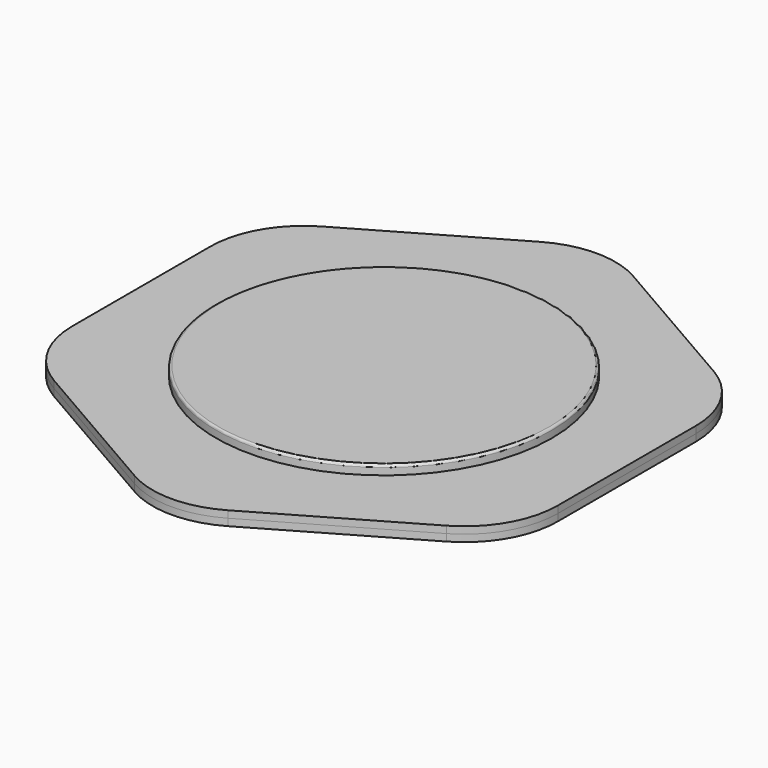
from build123d import *

# Parameters (mm, degrees)
F0_R      = 457.2
F1_DEPTH  = 6.35
F2_R      = 457.2
F2_R_2    = 12.7
F2_R_3    = 3.175
F2_R_4    = 74.6125
F3_DEPTH  = 19.05
F4_R      = 457.2
F4_R_2    = 12.7
F4_R_3    = 3.175
F4_R_4    = 15.875
F5_DEPTH  = 19.05
F6_R      = 74.6125
F6_R_2    = 3.175
F6_R_3    = 58.7375
F7_DEPTH  = 3.175
F9_R      = 457.2
F10_DEPTH = 19.05
F11_R     = 6.34999


# Not quite as in the source:
# - a fillet or chamfer is up to 0.001 mm smaller than in the source, because OpenCascade refuses the exact size


with BuildPart() as f1:
    # F0 (on Top) → F1 (new body)
    with BuildSketch(Plane.XY):
        Circle(F0_R)
    extrude(amount=-F1_DEPTH)

    # F11 (radius 6.35 in the source; OpenCascade refuses exactly that, so slightly less here)
    f11_edges = [f1.edges().sort_by_distance(p)[0] for p in [
        (-457.2, 0, 0),
    ]]
    fillet(f11_edges, radius=F11_R)


with BuildPart() as f3:
    # F2 (on face) → F3 (new body)
    with BuildSketch(Plane(origin=(0, 0, -6.35), x_dir=(1, 0, 0), z_dir=(0, 0, -1))):
        Circle(F2_R)
        with Locations((-291.8583239347, -291.8583239347)):
            Circle(F2_R_2, mode=Mode.SUBTRACT)
        with Locations((-260.427427511, -260.427427511)):
            Circle(F2_R_2, mode=Mode.SUBTRACT)
        with Locations((-228.9965310873, -228.9965310873)):
            Circle(F2_R_2, mode=Mode.SUBTRACT)
        with Locations((-157.9525867087, -381.331277044)):
            Circle(F2_R_3, mode=Mode.SUBTRACT)
        with Locations((-381.331277044, -157.9525867087)):
            Circle(F2_R_3, mode=Mode.SUBTRACT)
        with Locations((-197.5656346635, -197.5656346635)):
            Circle(F2_R_2, mode=Mode.SUBTRACT)
        with Locations((-166.1347382398, -166.1347382398)):
            Circle(F2_R_2, mode=Mode.SUBTRACT)
        with Locations((-134.703841816, -134.703841816)):
            Circle(F2_R_2, mode=Mode.SUBTRACT)
        with Locations((-103.2729453923, -103.2729453923)):
            Circle(F2_R_2, mode=Mode.SUBTRACT)
        with Locations((-71.8420489686, -71.8420489686)):
            Circle(F2_R_2, mode=Mode.SUBTRACT)
        with Locations((0, -412.75)):
            Circle(F2_R_2, mode=Mode.SUBTRACT)
        with Locations((0, -368.3)):
            Circle(F2_R_2, mode=Mode.SUBTRACT)
        with Locations((157.9525867087, -381.331277044)):
            Circle(F2_R_3, mode=Mode.SUBTRACT)
        with Locations((0, -323.85)):
            Circle(F2_R_2, mode=Mode.SUBTRACT)
        with Locations((0, -279.4)):
            Circle(F2_R_2, mode=Mode.SUBTRACT)
        with Locations((0, -234.95)):
            Circle(F2_R_2, mode=Mode.SUBTRACT)
        with Locations((291.8583239347, -291.8583239347)):
            Circle(F2_R_2, mode=Mode.SUBTRACT)
        with Locations((260.427427511, -260.427427511)):
            Circle(F2_R_2, mode=Mode.SUBTRACT)
        with Locations((228.9965310873, -228.9965310873)):
            Circle(F2_R_2, mode=Mode.SUBTRACT)
        with Locations((0, -190.5)):
            Circle(F2_R_2, mode=Mode.SUBTRACT)
        with Locations((0, -146.05)):
            Circle(F2_R_2, mode=Mode.SUBTRACT)
        with Locations((197.5656346635, -197.5656346635)):
            Circle(F2_R_2, mode=Mode.SUBTRACT)
        with Locations((166.1347382398, -166.1347382398)):
            Circle(F2_R_2, mode=Mode.SUBTRACT)
        with Locations((134.703841816, -134.703841816)):
            Circle(F2_R_2, mode=Mode.SUBTRACT)
        with Locations((0, -101.6)):
            Circle(F2_R_2, mode=Mode.SUBTRACT)
        with Locations((103.2729453923, -103.2729453923)):
            Circle(F2_R_2, mode=Mode.SUBTRACT)
        with Locations((71.8420489686, -71.8420489686)):
            Circle(F2_R_2, mode=Mode.SUBTRACT)
        with Locations((381.331277044, -157.9525867087)):
            Circle(F2_R_3, mode=Mode.SUBTRACT)
        with Locations((-412.75, 0)):
            Circle(F2_R_2, mode=Mode.SUBTRACT)
        with Locations((-368.3, 0)):
            Circle(F2_R_2, mode=Mode.SUBTRACT)
        with Locations((-323.85, 0)):
            Circle(F2_R_2, mode=Mode.SUBTRACT)
        with Locations((-279.4, 0)):
            Circle(F2_R_2, mode=Mode.SUBTRACT)
        with Locations((-234.95, 0)):
            Circle(F2_R_2, mode=Mode.SUBTRACT)
        with Locations((-381.331277044, 157.9525867087)):
            Circle(F2_R_3, mode=Mode.SUBTRACT)
        with Locations((-190.5, 0)):
            Circle(F2_R_2, mode=Mode.SUBTRACT)
        with Locations((-146.05, 0)):
            Circle(F2_R_2, mode=Mode.SUBTRACT)
        with Locations((-101.6, 0)):
            Circle(F2_R_2, mode=Mode.SUBTRACT)
        with Locations((-71.8420489686, 71.8420489686)):
            Circle(F2_R_2, mode=Mode.SUBTRACT)
        with Locations((-103.2729453923, 103.2729453923)):
            Circle(F2_R_2, mode=Mode.SUBTRACT)
        with Locations((-134.703841816, 134.703841816)):
            Circle(F2_R_2, mode=Mode.SUBTRACT)
        with Locations((-166.1347382398, 166.1347382398)):
            Circle(F2_R_2, mode=Mode.SUBTRACT)
        with Locations((-197.5656346635, 197.5656346635)):
            Circle(F2_R_2, mode=Mode.SUBTRACT)
        with Locations((-228.9965310873, 228.9965310873)):
            Circle(F2_R_2, mode=Mode.SUBTRACT)
        with Locations((-260.427427511, 260.427427511)):
            Circle(F2_R_2, mode=Mode.SUBTRACT)
        with Locations((-291.8583239347, 291.8583239347)):
            Circle(F2_R_2, mode=Mode.SUBTRACT)
        with Locations((-157.9525867087, 381.331277044)):
            Circle(F2_R_3, mode=Mode.SUBTRACT)
        Circle(F2_R_4, mode=Mode.SUBTRACT)
        with Locations((101.6, 0)):
            Circle(F2_R_2, mode=Mode.SUBTRACT)
        with Locations((0, 101.6)):
            Circle(F2_R_2, mode=Mode.SUBTRACT)
        with Locations((71.8420489686, 71.8420489686)):
            Circle(F2_R_2, mode=Mode.SUBTRACT)
        with Locations((103.2729453923, 103.2729453923)):
            Circle(F2_R_2, mode=Mode.SUBTRACT)
        with Locations((146.05, 0)):
            Circle(F2_R_2, mode=Mode.SUBTRACT)
        with Locations((190.5, 0)):
            Circle(F2_R_2, mode=Mode.SUBTRACT)
        with Locations((0, 146.05)):
            Circle(F2_R_2, mode=Mode.SUBTRACT)
        with Locations((0, 190.5)):
            Circle(F2_R_2, mode=Mode.SUBTRACT)
        with Locations((134.703841816, 134.703841816)):
            Circle(F2_R_2, mode=Mode.SUBTRACT)
        with Locations((166.1347382398, 166.1347382398)):
            Circle(F2_R_2, mode=Mode.SUBTRACT)
        with Locations((197.5656346635, 197.5656346635)):
            Circle(F2_R_2, mode=Mode.SUBTRACT)
        with Locations((234.95, 0)):
            Circle(F2_R_2, mode=Mode.SUBTRACT)
        with Locations((279.4, 0)):
            Circle(F2_R_2, mode=Mode.SUBTRACT)
        with Locations((323.85, 0)):
            Circle(F2_R_2, mode=Mode.SUBTRACT)
        with Locations((368.3, 0)):
            Circle(F2_R_2, mode=Mode.SUBTRACT)
        with Locations((412.75, 0)):
            Circle(F2_R_2, mode=Mode.SUBTRACT)
        with Locations((381.331277044, 157.9525867087)):
            Circle(F2_R_3, mode=Mode.SUBTRACT)
        with Locations((0, 234.95)):
            Circle(F2_R_2, mode=Mode.SUBTRACT)
        with Locations((0, 279.4)):
            Circle(F2_R_2, mode=Mode.SUBTRACT)
        with Locations((0, 323.85)):
            Circle(F2_R_2, mode=Mode.SUBTRACT)
        with Locations((0, 368.3)):
            Circle(F2_R_2, mode=Mode.SUBTRACT)
        with Locations((0, 412.75)):
            Circle(F2_R_2, mode=Mode.SUBTRACT)
        with Locations((157.9525867087, 381.331277044)):
            Circle(F2_R_3, mode=Mode.SUBTRACT)
        with Locations((228.9965310873, 228.9965310873)):
            Circle(F2_R_2, mode=Mode.SUBTRACT)
        with Locations((260.427427511, 260.427427511)):
            Circle(F2_R_2, mode=Mode.SUBTRACT)
        with Locations((291.8583239347, 291.8583239347)):
            Circle(F2_R_2, mode=Mode.SUBTRACT)
    extrude(amount=F3_DEPTH)


with BuildPart() as f5:
    # F4 (on face) → F5 (new body)
    with BuildSketch(Plane(origin=(0, 0, -25.4), x_dir=(1, 0, 0), z_dir=(0, 0, -1))):
        Circle(F4_R)
        with Locations((-291.8583239347, -291.8583239347)):
            Circle(F4_R_2, mode=Mode.SUBTRACT)
        with Locations((-260.427427511, -260.427427511)):
            Circle(F4_R_2, mode=Mode.SUBTRACT)
        with Locations((-228.9965310873, -228.9965310873)):
            Circle(F4_R_2, mode=Mode.SUBTRACT)
        with Locations((-157.9525867087, -381.331277044)):
            Circle(F4_R_3, mode=Mode.SUBTRACT)
        with Locations((-381.331277044, -157.9525867087)):
            Circle(F4_R_3, mode=Mode.SUBTRACT)
        with Locations((-197.5656346635, -197.5656346635)):
            Circle(F4_R_2, mode=Mode.SUBTRACT)
        with Locations((-166.1347382398, -166.1347382398)):
            Circle(F4_R_2, mode=Mode.SUBTRACT)
        with Locations((-134.703841816, -134.703841816)):
            Circle(F4_R_2, mode=Mode.SUBTRACT)
        with Locations((-103.2729453923, -103.2729453923)):
            Circle(F4_R_2, mode=Mode.SUBTRACT)
        with Locations((-71.8420489686, -71.8420489686)):
            Circle(F4_R_2, mode=Mode.SUBTRACT)
        with Locations((-33.3375, -57.7422437973)):
            Circle(F4_R_3, mode=Mode.SUBTRACT)
        with Locations((0, -412.75)):
            Circle(F4_R_2, mode=Mode.SUBTRACT)
        with Locations((0, -368.3)):
            Circle(F4_R_2, mode=Mode.SUBTRACT)
        with Locations((157.9525867087, -381.331277044)):
            Circle(F4_R_3, mode=Mode.SUBTRACT)
        with Locations((0, -323.85)):
            Circle(F4_R_2, mode=Mode.SUBTRACT)
        with Locations((0, -279.4)):
            Circle(F4_R_2, mode=Mode.SUBTRACT)
        with Locations((0, -234.95)):
            Circle(F4_R_2, mode=Mode.SUBTRACT)
        with Locations((291.8583239347, -291.8583239347)):
            Circle(F4_R_2, mode=Mode.SUBTRACT)
        with Locations((260.427427511, -260.427427511)):
            Circle(F4_R_2, mode=Mode.SUBTRACT)
        with Locations((228.9965310873, -228.9965310873)):
            Circle(F4_R_2, mode=Mode.SUBTRACT)
        with Locations((0, -190.5)):
            Circle(F4_R_2, mode=Mode.SUBTRACT)
        with Locations((0, -146.05)):
            Circle(F4_R_2, mode=Mode.SUBTRACT)
        with Locations((197.5656346635, -197.5656346635)):
            Circle(F4_R_2, mode=Mode.SUBTRACT)
        with Locations((166.1347382398, -166.1347382398)):
            Circle(F4_R_2, mode=Mode.SUBTRACT)
        with Locations((134.703841816, -134.703841816)):
            Circle(F4_R_2, mode=Mode.SUBTRACT)
        with Locations((0, -101.6)):
            Circle(F4_R_2, mode=Mode.SUBTRACT)
        with Locations((33.3375, -57.7422437973)):
            Circle(F4_R_3, mode=Mode.SUBTRACT)
        with Locations((103.2729453923, -103.2729453923)):
            Circle(F4_R_2, mode=Mode.SUBTRACT)
        with Locations((71.8420489686, -71.8420489686)):
            Circle(F4_R_2, mode=Mode.SUBTRACT)
        with Locations((381.331277044, -157.9525867087)):
            Circle(F4_R_3, mode=Mode.SUBTRACT)
        with Locations((-412.75, 0)):
            Circle(F4_R_2, mode=Mode.SUBTRACT)
        with Locations((-368.3, 0)):
            Circle(F4_R_2, mode=Mode.SUBTRACT)
        with Locations((-323.85, 0)):
            Circle(F4_R_2, mode=Mode.SUBTRACT)
        with Locations((-279.4, 0)):
            Circle(F4_R_2, mode=Mode.SUBTRACT)
        with Locations((-234.95, 0)):
            Circle(F4_R_2, mode=Mode.SUBTRACT)
        with Locations((-381.331277044, 157.9525867087)):
            Circle(F4_R_3, mode=Mode.SUBTRACT)
        with Locations((-190.5, 0)):
            Circle(F4_R_2, mode=Mode.SUBTRACT)
        with Locations((-146.05, 0)):
            Circle(F4_R_2, mode=Mode.SUBTRACT)
        with Locations((-101.6, 0)):
            Circle(F4_R_2, mode=Mode.SUBTRACT)
        with Locations((-66.675, 0)):
            Circle(F4_R_3, mode=Mode.SUBTRACT)
        with Locations((-71.8420489686, 71.8420489686)):
            Circle(F4_R_2, mode=Mode.SUBTRACT)
        with Locations((-103.2729453923, 103.2729453923)):
            Circle(F4_R_2, mode=Mode.SUBTRACT)
        with Locations((-33.3375, 57.7422437973)):
            Circle(F4_R_3, mode=Mode.SUBTRACT)
        with Locations((-134.703841816, 134.703841816)):
            Circle(F4_R_2, mode=Mode.SUBTRACT)
        with Locations((-166.1347382398, 166.1347382398)):
            Circle(F4_R_2, mode=Mode.SUBTRACT)
        with Locations((-197.5656346635, 197.5656346635)):
            Circle(F4_R_2, mode=Mode.SUBTRACT)
        with Locations((-228.9965310873, 228.9965310873)):
            Circle(F4_R_2, mode=Mode.SUBTRACT)
        with Locations((-260.427427511, 260.427427511)):
            Circle(F4_R_2, mode=Mode.SUBTRACT)
        with Locations((-291.8583239347, 291.8583239347)):
            Circle(F4_R_2, mode=Mode.SUBTRACT)
        with Locations((-157.9525867087, 381.331277044)):
            Circle(F4_R_3, mode=Mode.SUBTRACT)
        Circle(F4_R_4, mode=Mode.SUBTRACT)
        with Locations((66.675, 0)):
            Circle(F4_R_3, mode=Mode.SUBTRACT)
        with Locations((101.6, 0)):
            Circle(F4_R_2, mode=Mode.SUBTRACT)
        with Locations((33.3375, 57.7422437973)):
            Circle(F4_R_3, mode=Mode.SUBTRACT)
        with Locations((71.8420489686, 71.8420489686)):
            Circle(F4_R_2, mode=Mode.SUBTRACT)
        with Locations((103.2729453923, 103.2729453923)):
            Circle(F4_R_2, mode=Mode.SUBTRACT)
        with Locations((146.05, 0)):
            Circle(F4_R_2, mode=Mode.SUBTRACT)
        with Locations((190.5, 0)):
            Circle(F4_R_2, mode=Mode.SUBTRACT)
        with Locations((0, 146.05)):
            Circle(F4_R_2, mode=Mode.SUBTRACT)
        with Locations((0, 190.5)):
            Circle(F4_R_2, mode=Mode.SUBTRACT)
        with Locations((134.703841816, 134.703841816)):
            Circle(F4_R_2, mode=Mode.SUBTRACT)
        with Locations((166.1347382398, 166.1347382398)):
            Circle(F4_R_2, mode=Mode.SUBTRACT)
        with Locations((197.5656346635, 197.5656346635)):
            Circle(F4_R_2, mode=Mode.SUBTRACT)
        with Locations((234.95, 0)):
            Circle(F4_R_2, mode=Mode.SUBTRACT)
        with Locations((279.4, 0)):
            Circle(F4_R_2, mode=Mode.SUBTRACT)
        with Locations((323.85, 0)):
            Circle(F4_R_2, mode=Mode.SUBTRACT)
        with Locations((368.3, 0)):
            Circle(F4_R_2, mode=Mode.SUBTRACT)
        with Locations((412.75, 0)):
            Circle(F4_R_2, mode=Mode.SUBTRACT)
        with Locations((381.331277044, 157.9525867087)):
            Circle(F4_R_3, mode=Mode.SUBTRACT)
        with Locations((0, 234.95)):
            Circle(F4_R_2, mode=Mode.SUBTRACT)
        with Locations((0, 279.4)):
            Circle(F4_R_2, mode=Mode.SUBTRACT)
        with Locations((0, 323.85)):
            Circle(F4_R_2, mode=Mode.SUBTRACT)
        with Locations((0, 368.3)):
            Circle(F4_R_2, mode=Mode.SUBTRACT)
        with Locations((0, 412.75)):
            Circle(F4_R_2, mode=Mode.SUBTRACT)
        with Locations((157.9525867087, 381.331277044)):
            Circle(F4_R_3, mode=Mode.SUBTRACT)
        with Locations((228.9965310873, 228.9965310873)):
            Circle(F4_R_2, mode=Mode.SUBTRACT)
        with Locations((260.427427511, 260.427427511)):
            Circle(F4_R_2, mode=Mode.SUBTRACT)
        with Locations((291.8583239347, 291.8583239347)):
            Circle(F4_R_2, mode=Mode.SUBTRACT)
    extrude(amount=F5_DEPTH)


with BuildPart() as f7:
    # F6 (on face) → F7 (new body)
    with BuildSketch(Plane.XY.offset(-25.4)):
        Circle(F6_R)
        with Locations((-33.3375, -57.7422437973)):
            Circle(F6_R_2, mode=Mode.SUBTRACT)
        with Locations((33.3375, -57.7422437973)):
            Circle(F6_R_2, mode=Mode.SUBTRACT)
        with Locations((-66.675, 0)):
            Circle(F6_R_2, mode=Mode.SUBTRACT)
        with Locations((-33.3375, 57.7422437973)):
            Circle(F6_R_2, mode=Mode.SUBTRACT)
        Circle(F6_R_3, mode=Mode.SUBTRACT)
        with Locations((66.675, 0)):
            Circle(F6_R_2, mode=Mode.SUBTRACT)
        with Locations((33.3375, 57.7422437973)):
            Circle(F6_R_2, mode=Mode.SUBTRACT)
    extrude(amount=F7_DEPTH)


with BuildPart() as f8_1:
    # F8: copy of F5
    add(f5.part.moved(Location((0, 0, -19.05))))


with BuildPart() as f10:
    # F9 (on face) → F10 (new body)
    with BuildSketch(Plane.XY.offset(-25.4)):
        with BuildLine():
            Line((660.4, -234.6351493987), (660.4, 234.6351493987))
            ThreePointArc((660.4, 234.6351493987), (626.3704525612, 361.6351493987), (533.4, 454.6056019599))
            Line((533.4, 454.6056019599), (127, 689.2407513586))
            ThreePointArc((127, 689.2407513586), (0, 723.2702987973), (-127, 689.2407513586))
            Line((-127, 689.2407513586), (-533.4, 454.6056019599))
            ThreePointArc((-533.4, 454.6056019599), (-626.3704525612, 361.6351493987), (-660.4, 234.6351493987))
            Line((-660.4, 234.6351493987), (-660.4, -234.6351493987))
            ThreePointArc((-660.4, -234.6351493987), (-626.3704525612, -361.6351493987), (-533.4, -454.6056019599))
            Line((-533.4, -454.6056019599), (-127, -689.2407513586))
            ThreePointArc((-127, -689.2407513586), (0, -723.2702987973), (127, -689.2407513586))
            Line((127, -689.2407513586), (533.4, -454.6056019599))
            ThreePointArc((533.4, -454.6056019599), (626.3704525612, -361.6351493987), (660.4, -234.6351493987))
        make_face()
        Circle(F9_R, mode=Mode.SUBTRACT)
    extrude(amount=-F10_DEPTH)


with BuildPart() as f12_1:
    # F12: copy of F10
    add(f10.part.moved(Location((0, 0, -19.05))))


with BuildPart() as f13_1:
    # F13: copy of F7
    add(f7.part.moved(Location((0, 0, -41.275))))


with BuildPart() as f15:
    # F14 (on Front) → F15 (revolve)
    with BuildSketch(Plane.XZ):
        with BuildLine():
            Line((15.875, -3.175), (15.875, -25.4))
            Line((15.875, -25.4), (58.7375, -25.4))
            Line((58.7375, -25.4), (58.7375, -22.225))
            Line((58.7375, -22.225), (74.6125, -22.225))
            Line((74.6125, -22.225), (74.6125, -15.875))
            Line((74.6125, -15.875), (63.5910432677, -15.875))
            ThreePointArc((63.5910432677, -15.875), (49.7560065569, -13.9547684038), (36.966894044, -8.3392424886))
            Line((36.966894044, -8.3392424886), (28.575, -3.175))
            Line((28.575, -3.175), (15.875, -3.175))
        make_face()
    revolve(axis=Axis((0, 0, -4.5274426408), (0, 0, 1)))


with BuildPart() as f16_1:
    # F16: instance of F15
    add(f15.part.mirror(Plane(origin=(0, -0.0825638681, -44.45), x_dir=(1, 0, 0), z_dir=(0, 0, -1))))


solid = Compound([f1.part, f3.part, f5.part, f7.part, f8_1.part, f10.part, f12_1.part, f13_1.part, f15.part, f16_1.part])
